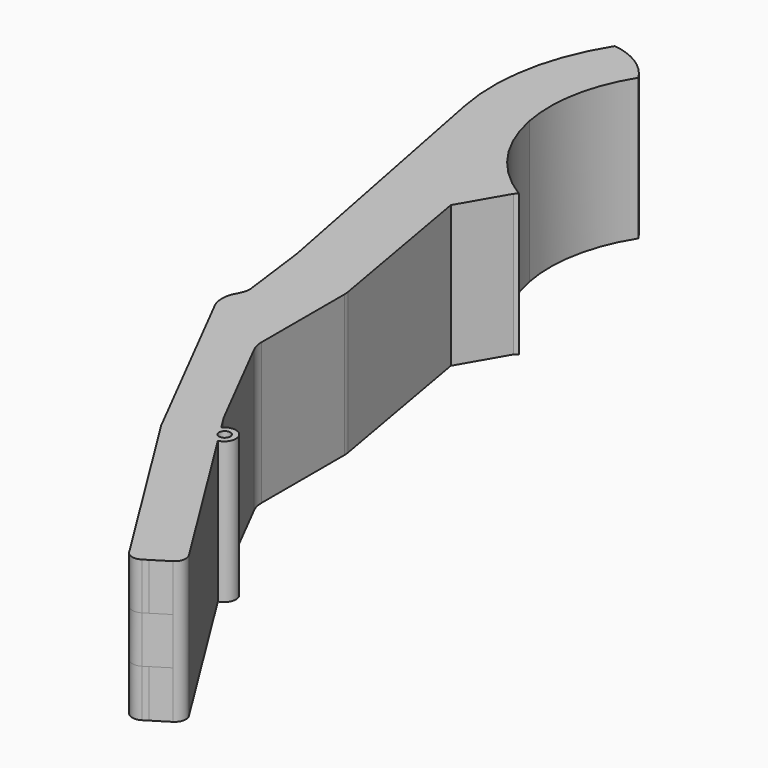
from build123d import *

# Parameters (mm, degrees)
F1_DEPTH  = 25
F2_DEPTH  = 25
F3_R      = 10.0351609687
F4_DEPTH  = 25
F5_W      = 5.021744368
F5_H      = 8.4
F5_W_2    = 5.524914672
F5_H_2    = 8.3
F6_DEPTH  = 28.7
F7_DEPTH  = 31.3
F8_W      = 20.0703219374
F8_H      = 8.3
F8_H_2    = 8.4
F9_DEPTH  = 25
F10_D     = 15
F11_DEPTH = 3
F12_DEPTH = 3
F13_DEPTH = 0.4
F15_DEPTH = 25
F16_R     = 5
F17_R     = 5
F18_R     = 5
F20_DEPTH = 25
F21_R     = 1
F22_DEPTH = 25
F24_DEPTH = 25
F25_R     = 2


with BuildPart() as f1:
    # F0 (on Top) → F1 (new body)
    with BuildSketch(Plane.XY):
        with BuildLine():
            Line((-46.5458918775, 92.7124905365), (-33.8341578848, 67.7643078592))
            Line((-33.8341578848, 67.7643078592), (-33.8341578848, 87.7643078592))
            Line((-33.8341578848, 87.7643078592), (-39.0436032148, 117.3085404495))
            ThreePointArc((-39.0436032148, 117.3085404495), (-50.1493049738, 127.7523979683), (-56.0863416463, 141.7938497088))
            Line((-56.0863416463, 141.7938497088), (-46.5458918775, 92.7124905365))
        make_face()
        Polygon((-26.4959632117, 42.4024048078), (0, 0), (0, 10), (-23.8463668905, 48.162164327), (-33.8341578848, 67.7643078592), (-46.5458918775, 92.7124905365), (-44.6555832012, 78.0426657754), align=None)
    extrude(amount=F1_DEPTH)

    # F0 (on Top) → F2 (join)
    with BuildSketch(Plane.XY):
        Polygon((-26.4959632117, 42.4024048078), (0, 0), (0, 10), (-23.8463668905, 48.162164327), (-33.8341578848, 67.7643078592), (-46.5458918775, 92.7124905365), (-44.6555832012, 78.0426657754), align=None)
        with BuildLine():
            Line((-46.5458918775, 92.7124905365), (-33.8341578848, 67.7643078592))
            Line((-33.8341578848, 67.7643078592), (-33.8341578848, 87.7643078592))
            Line((-33.8341578848, 87.7643078592), (-39.0436032148, 117.3085404495))
            ThreePointArc((-39.0436032148, 117.3085404495), (-50.1493049738, 127.7523979683), (-56.0863416463, 141.7938497088))
            Line((-56.0863416463, 141.7938497088), (-46.5458918775, 92.7124905365))
        make_face()
        with BuildLine():
            ThreePointArc((-51.0571508097, 168.5508889923), (-56.1292788842, 155.6530772369), (-56.0863416463, 141.7938497088))
            ThreePointArc((-56.0863416463, 141.7938497088), (-50.1493049738, 127.7523979683), (-39.0436032148, 117.3085404495))
            ThreePointArc((-39.0436032148, 117.3085404495), (-37.3018340244, 121.656861024), (-34.4069625383, 125.3394376776))
            ThreePointArc((-34.4069625383, 125.3394376776), (-34.1290622054, 125.5985630521), (-33.8452613454, 125.8512122687))
            ThreePointArc((-33.8452613454, 125.8512122687), (-46.0977457681, 142.6841841118), (-42.6035759811, 163.2088788258))
            ThreePointArc((-42.6035759811, 163.2088788258), (-46.2302574516, 166.8295340113), (-51.0571508097, 168.5508889923))
        make_face()
        with BuildLine():
            ThreePointArc((-34.4069625383, 125.3394376776), (-37.3018340244, 121.656861024), (-39.0436032148, 117.3085404495))
            Line((-39.0436032148, 117.3085404495), (-34.4069625383, 125.3394376776))
        make_face()
        with BuildLine():
            ThreePointArc((-46.2700698118, 143.7019396626), (-46.3013690244, 153.8058664235), (-42.6035759811, 163.2088788258))
            ThreePointArc((-42.6035759811, 163.2088788258), (-46.0977457681, 142.6841841118), (-33.8452613454, 125.8512122687))
            ThreePointArc((-33.8452613454, 125.8512122687), (-41.9417428936, 133.4651840398), (-46.2700698118, 143.7019396626))
        make_face()
    extrude(amount=F2_DEPTH)

    # F3 (on Top) → F4 (join)
    with BuildSketch(Plane.XY):
        Circle(F3_R)
    extrude(amount=F4_DEPTH)

    # F5 (on face) → F6 (join)
    with BuildSketch(Plane(origin=(0, 0, 0), x_dir=(0.5299192642, -0.8480480962, 0), z_dir=(-0.8480480962, -0.5299192642, 0))):
        with Locations((-12.5460331527, 4.2)):
            Rectangle(F5_W, F5_H)
        with Locations((-12.7976183047, 20.85)):
            Rectangle(F5_W_2, F5_H_2)
    extrude(amount=F6_DEPTH)

    # F7 (cut, symmetric): faces of the model
    f7_faces = [f1.faces().sort_by_distance(p)[0] for p in [
        (-17.4873152969, 0.9059577124, 20.85),
        (-17.4873152969, 0.9059577124, 4.2),
    ]]
    extrude(f7_faces, amount=F7_DEPTH, both=True, mode=Mode.SUBTRACT)

    # F8 (on face) → F9 (cut)
    with BuildSketch(Plane(origin=(0, 0, 0), x_dir=(0.5299192642, -0.8480480962, 0), z_dir=(-0.8480480962, -0.5299192642, 0))):
        with Locations((0, 20.85)):
            Rectangle(F8_W, F8_H)
        with Locations((0, 4.2)):
            Rectangle(F8_W, F8_H_2)
    extrude(amount=-F9_DEPTH, mode=Mode.SUBTRACT)

    # F10 (through all)
    with Locations(Plane(origin=(0, 0, 0), x_dir=(1, 0, 0), z_dir=(0, 0, -1))):
        with Locations((0, 0)):
            Hole(F10_D / 2)

    # F11 (add): a face of the model
    f11_faces = [f1.faces().sort_by_distance(p)[0] for p in [
        (-15.9068941643, 25.456351981, 12.5),
    ]]
    extrude(f11_faces, amount=F11_DEPTH)

    # F12 (add): a face of the model
    f12_faces = [f1.faces().sort_by_distance(p)[0] for p in [
        (-35.5757732065, 60.2225352916, 12.5),
    ]]
    extrude(f12_faces, amount=F12_DEPTH)

    # F13 (add): a face of the model
    f13_faces = [f1.faces().sort_by_distance(p)[0] for p in [
        (-27.7680353559, 41.6075259115, 12.5),
    ]]
    extrude(f13_faces, amount=F13_DEPTH)

    # F14 (on face) → F15 (join)
    with BuildSketch(Plane.XY.offset(25)):
        with BuildLine():
            ThreePointArc((-44.9484246095, 80.3152745808), (-45.6553028657, 78.1815440804), (-47.3286027738, 76.6806942761))
            Line((-47.3286027738, 76.6806942761), (-44.6555832012, 78.0426657754))
            Line((-44.6555832012, 78.0426657754), (-44.9484246095, 80.3152745808))
        make_face()
        with BuildLine():
            Line((-44.6555832012, 78.0426657754), (-47.3286027738, 76.6806942761))
            Line((-47.3286027738, 76.6806942761), (-29.2321155859, 41.1643384084))
            Line((-29.2321155859, 41.1643384084), (-29.2520752058, 41.1518662536))
            Line((-29.2520752058, 41.1518662536), (-7.8619694055, 6.9205413615))
            Line((-7.8619694055, 6.9205413615), (-0.8238548855, 11.3184434202))
            Line((-0.8238548855, 11.3184434202), (-23.8463668905, 48.162164327))
            Line((-23.8463668905, 48.162164327), (-33.8341578848, 67.7643078592))
            Line((-33.8341578848, 67.7643078592), (-33.8341578848, 87.7643078592))
            Line((-33.8341578848, 87.7643078592), (-39.0436032148, 117.3085404495))
            Line((-39.0436032148, 117.3085404495), (-34.4069625383, 125.3394376776))
            ThreePointArc((-34.4069625383, 125.3394376776), (-34.1290622054, 125.5985630521), (-33.8452613454, 125.8512122687))
            ThreePointArc((-33.8452613454, 125.8512122687), (-46.0541257293, 142.6944106077), (-42.6035759811, 163.2088788258))
            ThreePointArc((-42.6035759811, 163.2088788258), (-46.2302574516, 166.8295340113), (-51.0571508097, 168.5508889923))
            ThreePointArc((-51.0571508097, 168.5508889923), (-56.1292788842, 155.6530772369), (-56.0863416463, 141.7938497088))
            Line((-56.0863416463, 141.7938497088), (-46.5458918775, 92.7124905365))
            Line((-46.5458918775, 92.7124905365), (-45.1575485807, 81.9381904826))
            ThreePointArc((-45.1575485807, 81.9381904826), (-44.9764120983, 81.1365996867), (-44.9484246095, 80.3152745808))
            Line((-44.9484246095, 80.3152745808), (-44.6555832012, 78.0426657754))
        make_face()
    extrude(amount=-F15_DEPTH)

    # F16
    f16_edges = [f1.edges().sort_by_distance(p)[0] for p in [
        (-47.328603, 76.680694, 12.5),
    ]]
    fillet(f16_edges, radius=F16_R)

    # F17
    f17_edges = [f1.edges().sort_by_distance(p)[0] for p in [
        (-33.834158, 67.764308, 12.5),
    ]]
    fillet(f17_edges, radius=F17_R)

    # F18
    f18_edges = [f1.edges().sort_by_distance(p)[0] for p in [
        (-33.834158, 87.764308, 12.5),
    ]]
    fillet(f18_edges, radius=F18_R)

    # F19 (on face) → F20 (join)
    with BuildSketch(Plane.XY.offset(25)):
        with BuildLine():
            Line((-22.2566090978, 45.6180200386), (-20.1369320409, 42.2258276539))
            ThreePointArc((-20.1369320409, 42.2258276539), (-18.8920264045, 45.3620878389), (-22.2566090978, 45.6180200386))
        make_face()
    extrude(amount=-F20_DEPTH)

    # F21 (on face) → F22 (cut)
    with BuildSketch(Plane.XY.offset(25)):
        with Locations((-20.5885408694, 44.3029189806)):
            Circle(F21_R)
    extrude(amount=-F22_DEPTH, mode=Mode.SUBTRACT)

    # F23 (on face) → F24 (cut)
    with BuildSketch(Plane.XY.offset(16.7)):
        Polygon((-21.581498906, -1.6523721461), (-21.581498906, -2.9845223762), (2.6676976122, -15.5032956973), (23.1070481241, 1.1343396036), (-0.8238548855, 11.3184434202), align=None)
    extrude(amount=-F24_DEPTH, mode=Mode.SUBTRACT)

    # F25
    f25_edges = [f1.edges().sort_by_distance(p)[0] for p in [
        (-0.823855, 11.318443, 12.5),
        (-7.861969, 6.920541, 12.5),
    ]]
    fillet(f25_edges, radius=F25_R)


solid = f1.part
